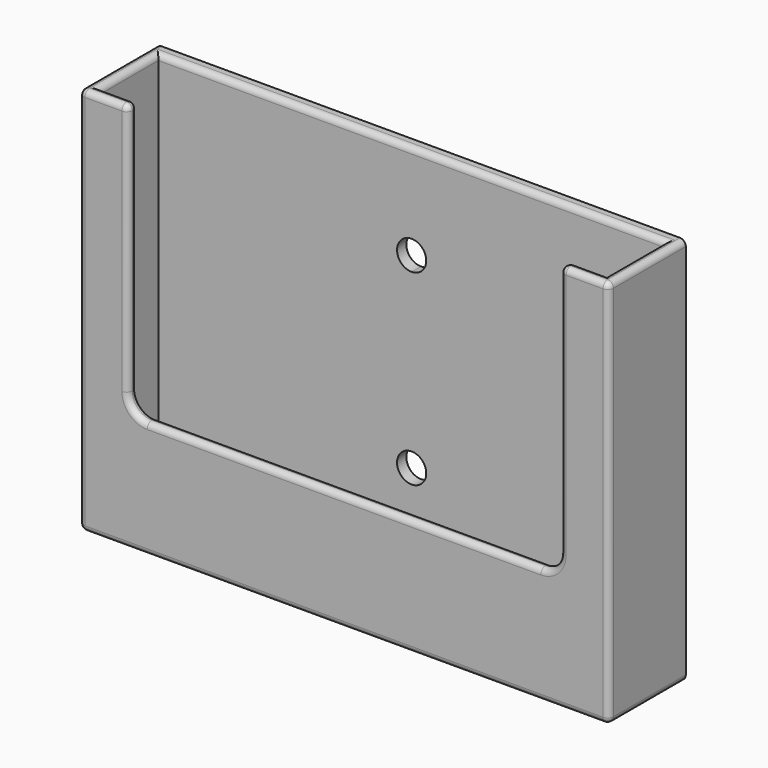
from build123d import *

# Parameters (mm, degrees)
F1_DEPTH = 1.2
F3_DEPTH = 7.5
F5_DEPTH = 1.2
F6_R     = 0.59999


# Not quite as in the source:
# - a fillet or chamfer is up to 0.001 mm smaller than in the source, because OpenCascade refuses the exact size


with BuildPart() as f1:
    # F0 (on Front) → F1 (new body)
    with BuildSketch(Plane.XZ):
        Polygon((-28.9807687655, 0), (-30.1807687655, 0), (-30.1807687655, -40), (24.3192312345, -40), (24.3192312345, 0), (23.1192312345, 0), (23.1192312345, -38.8), (-28.9807687655, -38.8), align=None)
        Polygon((-2.9307687655, -19.4), (-28.9807687655, 0), (-28.9807687655, -38.8), align=None)
        with BuildLine():
            Line((23.1192312345, 0), (-28.9807687655, 0))
            Line((-28.9807687655, 0), (-2.9307687655, -19.4))
            Line((-2.9307687655, -19.4), (-2.9307687655, -11.2695819765))
            ThreePointArc((-2.9307687655, -11.2695819765), (-3.9914289373, -8.7089218048), (-1.4307687655, -9.7695819765))
            Line((-1.4307687655, -9.7695819765), (3.4249790478, -9.7695819765))
            Line((3.4249790478, -9.7695819765), (3.4249790478, -14.6667367532))
            Line((3.4249790478, -14.6667367532), (23.1192312345, 0))
        make_face()
        Polygon((23.1192312345, -38.8), (23.1192312345, 0), (3.4249790478, -14.6667367532), (3.4249790478, -19.4), (3.3088028431, -19.4), (3.3088028431, -24.0467443074), align=None)
        with BuildLine():
            Line((-2.9307687655, -19.4), (-28.9807687655, -38.8))
            Line((-28.9807687655, -38.8), (23.1192312345, -38.8))
            Line((23.1192312345, -38.8), (3.3088028431, -24.0467443074))
            Line((3.3088028431, -24.0467443074), (3.3088028431, -29.0304180235))
            Line((3.3088028431, -29.0304180235), (-1.4307687655, -29.0304180235))
            ThreePointArc((-1.4307687655, -29.0304180235), (-3.9914289373, -30.0910781952), (-2.9307687655, -27.5304180235))
            Line((-2.9307687655, -27.5304180235), (-2.9307687655, -19.4))
        make_face()
        with BuildLine():
            Line((3.3088028431, -24.0467443074), (-2.9307687655, -19.4))
            Line((-2.9307687655, -19.4), (-2.9307687655, -27.5304180235))
            ThreePointArc((-2.9307687655, -27.5304180235), (-1.8701085937, -27.9697578517), (-1.4307687655, -29.0304180235))
            Line((-1.4307687655, -29.0304180235), (3.3088028431, -29.0304180235))
            Line((3.3088028431, -29.0304180235), (3.3088028431, -24.0467443074))
        make_face()
        Polygon((3.3088028431, -19.4), (-2.9307687655, -19.4), (3.3088028431, -24.0467443074), align=None)
        Polygon((3.4249790478, -14.6667367532), (-2.9307687655, -19.4), (3.3088028431, -19.4), (3.4249790478, -19.4), align=None)
        with BuildLine():
            Line((-2.9307687655, -11.2695819765), (-2.9307687655, -19.4))
            Line((-2.9307687655, -19.4), (3.4249790478, -14.6667367532))
            Line((3.4249790478, -14.6667367532), (3.4249790478, -9.7695819765))
            Line((3.4249790478, -9.7695819765), (-1.4307687655, -9.7695819765))
            ThreePointArc((-1.4307687655, -9.7695819765), (-1.8701085937, -10.8302421483), (-2.9307687655, -11.2695819765))
        make_face()
    extrude(amount=F1_DEPTH)

    # F2 (on face) → F3 (join)
    with BuildSketch(Plane.XZ.offset(1.2)):
        Polygon((-30.1807687655, 0), (-30.1807687655, -40), (24.3192312345, -40), (24.3192312345, 0), (23.1192312345, 0), (23.1192312345, -38.8), (-28.9807687655, -38.8), (-28.9807687655, 0), align=None)
    extrude(amount=F3_DEPTH)

    # F4 (on face) → F5 (join)
    with BuildSketch(Plane.XZ.offset(8.7)):
        with BuildLine():
            Line((-25.1807687655, 0), (-28.9807687655, 0))
            Line((-28.9807687655, 0), (-28.9807687655, -38.8))
            Line((-28.9807687655, -38.8), (23.1192312345, -38.8))
            Line((23.1192312345, -38.8), (23.1192312345, 0))
            Line((23.1192312345, 0), (19.3192312345, 0))
            Line((19.3192312345, 0), (19.3192312345, -26))
            ThreePointArc((19.3192312345, -26), (18.7334447969, -27.4142135624), (17.3192312345, -28))
            Line((17.3192312345, -28), (-23.1807687655, -28))
            ThreePointArc((-23.1807687655, -28), (-24.5949823279, -27.4142135624), (-25.1807687655, -26))
            Line((-25.1807687655, -26), (-25.1807687655, 0))
        make_face()
        Polygon((-30.1807687655, 0), (-30.1807687655, -40), (24.3192312345, -40), (24.3192312345, 0), (23.1192312345, 0), (23.1192312345, -38.8), (-28.9807687655, -38.8), (-28.9807687655, 0), align=None)
    extrude(amount=F5_DEPTH)

    # F6 (radius 0.6 in the source; OpenCascade refuses exactly that, so slightly less here)
    f6_edges = [f1.edges().sort_by_distance(p)[0] for p in [
        (-30.180769, -4.95, -40),
        (24.319231, -4.95, -40),
        (-30.180769, -4.95, 0),
        (-27.680769, -9.9, 0),
        (24.319231, -4.95, 0),
        (21.819231, -9.9, 0),
        (-2.930769, -9.9, -40),
        (24.319231, -9.9, -20),
        (-30.180769, -9.9, -20),
        (-25.180769, -9.9, -13),
        (-2.930769, -8.7, -28),
        (19.319231, -8.7, -13),
        (-27.080769, -8.7, 0),
        (-28.980769, -4.95, 0),
        (23.119231, -4.95, 0),
        (21.219231, -8.7, 0),
        (19.319231, -9.3, 0),
        (-25.180769, -9.3, 0),
        (-2.930769, -1.2, 0),
    ]]
    fillet(f6_edges, radius=F6_R)


solid = f1.part
